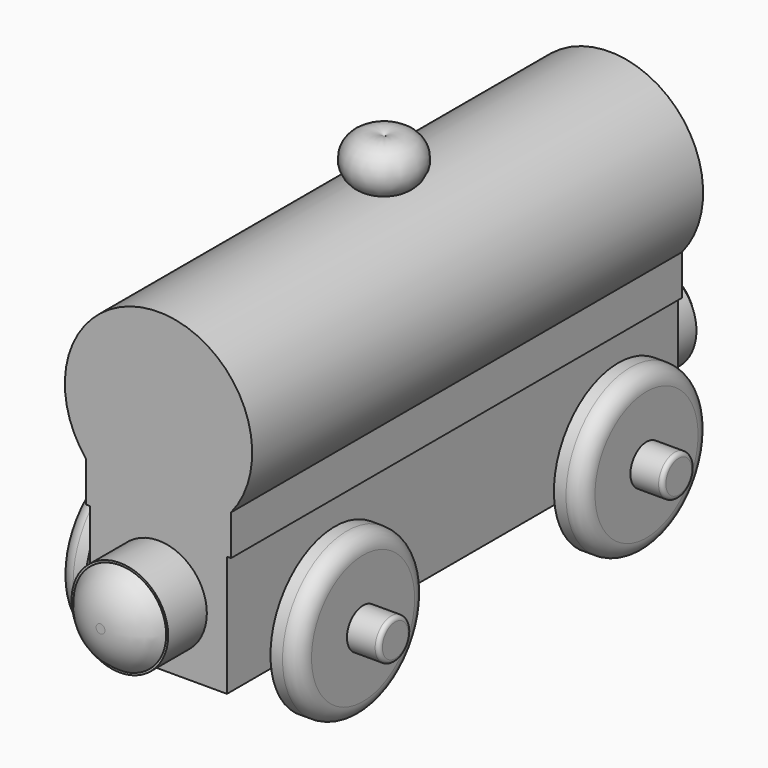
from build123d import *

# Parameters (mm, degrees)
F1_DEPTH  = 35
F2_W      = 18
F2_H      = 5
F3_DEPTH  = 70
F5_W      = 17
F5_H      = 70
F6_DEPTH  = 15
F7_R      = 6
F8_DEPTH  = 6
F9_R      = 6
F10_DEPTH = 6
F13_R     = 4
F14_DEPTH = 3
F15_R     = 4
F16_DEPTH = 3
F17_R     = 4
F18_DEPTH = 3
F19_R     = 4
F20_DEPTH = 3
F21_R     = 10
F22_DEPTH = 3.5
F23_R     = 10
F24_DEPTH = 3.5
F25_R     = 10
F26_DEPTH = 3.5
F27_R     = 10
F28_DEPTH = 3.5
F29_R     = 2.5
F30_DEPTH = 4
F31_R     = 2.5
F32_DEPTH = 4
F33_R     = 2.5
F34_DEPTH = 4
F35_R     = 2.5
F36_DEPTH = 4
F37_R     = 2
F38_R     = 2
F39_R     = 2
F40_R     = 2
F41_R     = 5.75
F42_DEPTH = 3
F44_R     = 5.75
F45_DEPTH = 3
F47_R     = 0.5
F48_R     = 0.5
F49_R     = 0.5
F50_R     = 0.5


# Not quite as in the source:
# - a fillet or chamfer that OpenCascade refuses, or shapes differently, is made with other operations: its cross-section is extruded or revolved along the edge and cut away or added


with BuildPart() as f1:
    # F0 (on Front) → F1 (new body, symmetric)
    with BuildSketch(Plane.XZ):
        with BuildLine():
            ThreePointArc((9, -7.3684210526), (0, 11.6315789474), (-9, -7.3684210526))
            Line((-9, -7.3684210526), (9, -7.3684210526))
        make_face()
    extrude(amount=F1_DEPTH, both=True)

    # F2 (on face) → F3 (join)
    with BuildSketch(Plane.XZ.offset(35)):
        with Locations((0, -9.8684210526)):
            Rectangle(F2_W, F2_H)
    extrude(amount=-F3_DEPTH)

    # F4: union 

    # F5 (on face) → F6 (join)
    with BuildSketch(Plane(origin=(0, 0, -12.3684210526), x_dir=(1, 0, 0), z_dir=(0, 0, -1))):
        Rectangle(F5_W, F5_H)
    extrude(amount=F6_DEPTH)

    # F7 (on face) → F8 (join)
    with BuildSketch(Plane.XZ.offset(35)):
        with Locations((0, -19.3684210526)):
            Circle(F7_R)
    extrude(amount=F8_DEPTH)

    # F9 (on face) → F10 (join)
    with BuildSketch(Plane(origin=(0, 35, 0), x_dir=(-1, 0, 0), z_dir=(0, 1, 0))):
        with Locations((0, -19.3684210526)):
            Circle(F9_R)
    extrude(amount=F10_DEPTH)

    # F11 (on Front) → F12 (revolve)
    with BuildSketch(Plane.XZ):
        with BuildLine():
            ThreePointArc((0, 16.6315789474), (-4.5, 14.1315789474), (0, 11.6315789474))
            Line((0, 11.6315789474), (0, 16.6315789474))
        make_face()
    revolve(axis=Axis((0, 0, -4.5549966032), (0, 0, -1)))

    # F13 (on face) → F14 (join)
    with BuildSketch(Plane.YZ.offset(8.5)):
        with Locations((-22, -23.3684210526)):
            Circle(F13_R)
    extrude(amount=F14_DEPTH)

    # F15 (on face) → F16 (join)
    with BuildSketch(Plane.YZ.offset(8.5)):
        with Locations((22, -23.3684210526)):
            Circle(F15_R)
    extrude(amount=F16_DEPTH)

    # F17 (on face) → F18 (join)
    with BuildSketch(Plane(origin=(-8.5, 0, 0), x_dir=(0, -1, 0), z_dir=(-1, 0, 0))):
        with Locations((22, -23.3684210526)):
            Circle(F17_R)
    extrude(amount=F18_DEPTH)

    # F19 (on face) → F20 (join)
    with BuildSketch(Plane(origin=(-8.5, 0, 0), x_dir=(0, -1, 0), z_dir=(-1, 0, 0))):
        with Locations((-22, -23.3684210526)):
            Circle(F19_R)
    extrude(amount=F20_DEPTH)

    # F21 (on face) → F22 (join)
    with BuildSketch(Plane(origin=(-11.5, 0, 0), x_dir=(0, -1, 0), z_dir=(-1, 0, 0))):
        with Locations((-22, -23.3684210526)):
            Circle(F21_R)
    extrude(amount=F22_DEPTH)

    # F23 (on face) → F24 (join)
    with BuildSketch(Plane(origin=(-11.5, 0, 0), x_dir=(0, -1, 0), z_dir=(-1, 0, 0))):
        with Locations((22, -23.3684210526)):
            Circle(F23_R)
    extrude(amount=F24_DEPTH)

    # F25 (on face) → F26 (join)
    with BuildSketch(Plane.YZ.offset(11.5)):
        with Locations((-22, -23.3684210526)):
            Circle(F25_R)
    extrude(amount=F26_DEPTH)

    # F27 (on face) → F28 (join)
    with BuildSketch(Plane.YZ.offset(11.5)):
        with Locations((22, -23.3684210526)):
            Circle(F27_R)
    extrude(amount=F28_DEPTH)

    # F29 (on face) → F30 (join)
    with BuildSketch(Plane.YZ.offset(15)):
        with Locations((-22, -23.3684210526)):
            Circle(F29_R)
    extrude(amount=F30_DEPTH)

    # F31 (on face) → F32 (join)
    with BuildSketch(Plane.YZ.offset(15)):
        with Locations((22, -23.3684210526)):
            Circle(F31_R)
    extrude(amount=F32_DEPTH)

    # F33 (on face) → F34 (join)
    with BuildSketch(Plane(origin=(-15, 0, 0), x_dir=(0, -1, 0), z_dir=(-1, 0, 0))):
        with Locations((-22, -23.3684210526)):
            Circle(F33_R)
    extrude(amount=F34_DEPTH)

    # F35 (on face) → F36 (join)
    with BuildSketch(Plane(origin=(-15, 0, 0), x_dir=(0, -1, 0), z_dir=(-1, 0, 0))):
        with Locations((22, -23.3684210526)):
            Circle(F35_R)
    extrude(amount=F36_DEPTH)

    # F37
    f37_edges = [f1.edges().sort_by_distance(p)[0] for p in [
        (-15, 32, -23.368421),
    ]]
    fillet(f37_edges, radius=F37_R)

    # F38
    f38_edges = [f1.edges().sort_by_distance(p)[0] for p in [
        (-15, -12, -23.368421),
    ]]
    fillet(f38_edges, radius=F38_R)

    # F39
    f39_edges = [f1.edges().sort_by_distance(p)[0] for p in [
        (15, -32, -23.368421),
    ]]
    fillet(f39_edges, radius=F39_R)

    # F40
    f40_edges = [f1.edges().sort_by_distance(p)[0] for p in [
        (15, 12, -23.368421),
    ]]
    fillet(f40_edges, radius=F40_R)

    # F41 (on face) → F42 (join)
    with BuildSketch(Plane(origin=(0, 41, 0), x_dir=(-1, 0, 0), z_dir=(0, 1, 0))):
        with Locations((0, -19.3684210526)):
            Circle(F41_R)
    extrude(amount=F42_DEPTH)

    # F43: fillet of radius 6 on 1 edges, made by hand

    # F43_s1 → F43_t2 (revolve, cut)
    with BuildSketch(Plane.XY.offset(-19.3684210526)):
        with BuildLine():
            ThreePointArc((-5.75, 41), (-3.5538475773, 43.1961524227), (-0.5538475773, 44))
            Line((-0.5538475773, 44), (-5.75, 44))
            Line((-5.75, 44), (-5.75, 41))
        make_face()
    revolve(axis=Axis((0, 44, -19.3684210526), (0, 1, 0)), mode=Mode.SUBTRACT)

    # F44 (on face) → F45 (join)
    with BuildSketch(Plane.XZ.offset(41)):
        with Locations((0, -19.3684210526)):
            Circle(F44_R)
    extrude(amount=F45_DEPTH)

    # F46: fillet of radius 6 on 1 edges, made by hand

    # F46_s1 → F46_t2 (revolve, cut)
    with BuildSketch(Plane.XY.offset(-19.3684210526)):
        with BuildLine():
            ThreePointArc((5.75, -41), (3.5538475773, -43.1961524227), (0.5538475773, -44))
            Line((0.5538475773, -44), (5.75, -44))
            Line((5.75, -44), (5.75, -41))
        make_face()
    revolve(axis=Axis((0, -44, -19.3684210526), (0, -1, 0)), mode=Mode.SUBTRACT)

    # F47
    f47_edges = [f1.edges().sort_by_distance(p)[0] for p in [
        (-19, -19.5, -23.368421),
    ]]
    fillet(f47_edges, radius=F47_R)

    # F48
    f48_edges = [f1.edges().sort_by_distance(p)[0] for p in [
        (-19, 24.5, -23.368421),
    ]]
    fillet(f48_edges, radius=F48_R)

    # F49
    f49_edges = [f1.edges().sort_by_distance(p)[0] for p in [
        (19, -24.5, -23.368421),
    ]]
    fillet(f49_edges, radius=F49_R)

    # F50
    f50_edges = [f1.edges().sort_by_distance(p)[0] for p in [
        (19, 19.5, -23.368421),
    ]]
    fillet(f50_edges, radius=F50_R)


solid = f1.part
